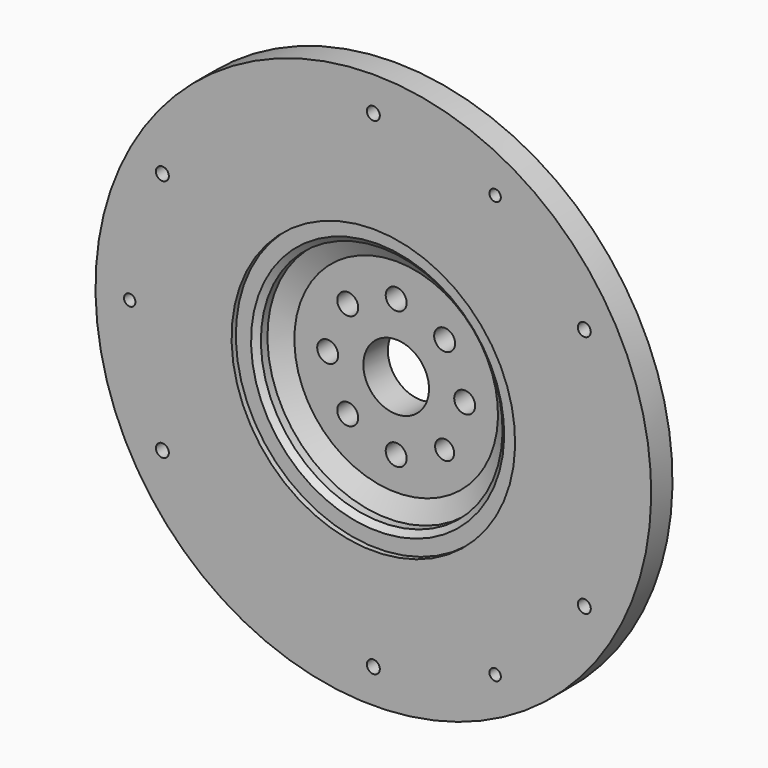
from build123d import *

# Parameters (mm, degrees)
F2_R      = 5.5
F2_R_2    = 5
F3_DEPTH  = 16.101
F4_R      = 3.4
F4_R_2    = 3
F5_DEPTH  = 31.101
F10_D     = 4
F10_DEPTH = 9
F10_TIP   = 1.2017212381


with BuildPart() as f1:
    # F0 (on Right) → F1 (revolve)
    with BuildSketch(Plane.YZ):
        Polygon((-31.1, 146), (-31.1, 74.5), (-28.3, 74.5), (-28.3, 66.5), (-25.6, 63.5), (-21.3, 63.5), (-16.1, 53.5), (-16.1, 17.25), (0, 17.25), (0, 44), (-15, 75), (-15, 112), (-8.5, 112), (-8.5, 135), (-17.1, 135), (-17.1, 146), align=None)
    revolve(axis=Axis((0, -8.05, 0), (0, -1, 0)))

    # F2 (on face) → F3 (cut, through all)
    with BuildSketch(Plane.XZ.offset(16.1)):
        with Locations((0, 36)):
            Circle(F2_R)
        with Locations((-25.4558441227, 25.4558441227)):
            Circle(F2_R)
        with Locations((-36, 0)):
            Circle(F2_R)
        with Locations((-25.4558441227, -25.4558441227)):
            Circle(F2_R)
        with Locations((0, -36)):
            Circle(F2_R)
        with Locations((25.4558441227, -25.4558441227)):
            Circle(F2_R_2)
        with Locations((36, 0)):
            Circle(F2_R)
        with Locations((25.4558441227, 25.4558441227)):
            Circle(F2_R)
    extrude(amount=-F3_DEPTH, mode=Mode.SUBTRACT)

    # F4 (on face) → F5 (cut, through all)
    with BuildSketch(Plane.XZ.offset(31.1)):
        with Locations((0, 128)):
            Circle(F4_R)
        with Locations((-110.8512516844, 64)):
            Circle(F4_R)
        with Locations((-110.8512516844, -64)):
            Circle(F4_R)
        with Locations((0, -128)):
            Circle(F4_R)
        with Locations((110.8512516844, -64)):
            Circle(F4_R)
        with Locations((110.8512516844, 64)):
            Circle(F4_R)
        with Locations((-128, 0)):
            Circle(F4_R_2)
        with Locations((64, -110.8512516844)):
            Circle(F4_R_2)
        with Locations((64, 110.8512516844)):
            Circle(F4_R_2)
    extrude(amount=-F5_DEPTH, mode=Mode.SUBTRACT)

    # F10 (one way)
    with BuildSketch(Plane(origin=(-32.8428539342, 0, -142.2580294586), x_dir=(0.9743700648, 0, -0.2249510543), z_dir=(-0.2249510543, 0, -0.9743700648))):
        with Locations((0, 25)):
            Circle(F10_D / 2)
    extrude(amount=-F10_DEPTH, mode=Mode.SUBTRACT)
    with Locations(Plane(origin=(-32.8428539342, 0, -142.2580294586), x_dir=(0.9743700648, 0, -0.2249510543), z_dir=(-0.2249510543, 0, -0.9743700648))):
        with Locations((0, 25)):
            with Locations((0, 0, -(F10_DEPTH + F10_TIP / 2))):  # 118° drill point
                Cone(0, F10_D / 2, F10_TIP, mode=Mode.SUBTRACT)


solid = f1.part
